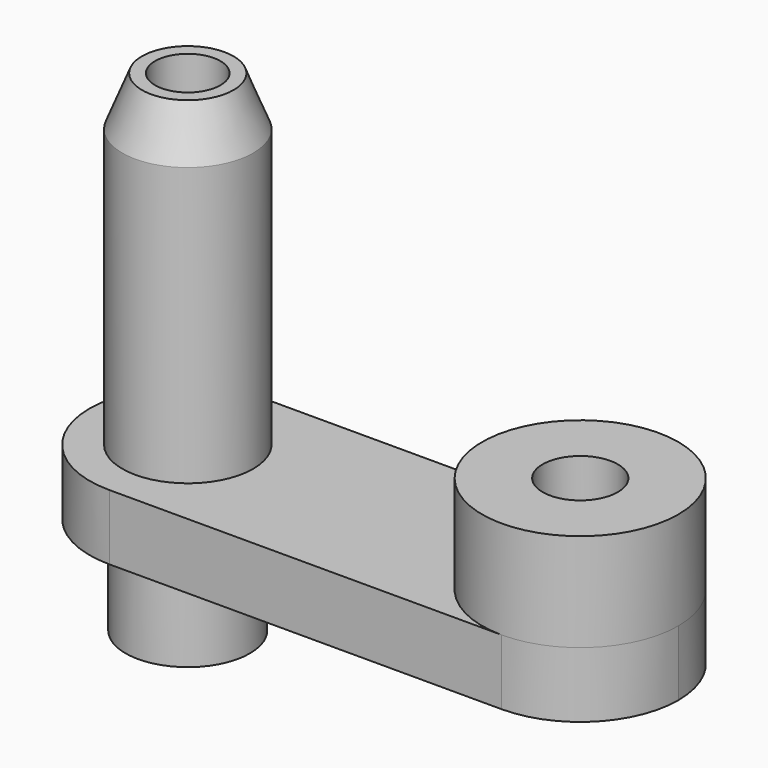
from build123d import *

# Parameters (mm, degrees)
F0_W      = 18
F0_H      = 6
F1_DEPTH  = 2
F2_R      = 3
F2_R_2    = 2
F3_DEPTH  = 10
F4_R      = 1
F4_R_2    = 1.15
F5_DEPTH  = 20
F6_SIZE2  = 1.5
F6_SIZE   = 0.6
F7_W      = 11.6012076614
F7_H      = 11.8295210414
F8_DEPTH  = 7
F9_R      = 2.9999
F10_R     = 1.9
F10_R_2   = 1
F11_DEPTH = 3


# Not quite as in the source:
# - a fillet or chamfer is up to 0.001 mm smaller than in the source, because OpenCascade refuses the exact size


with BuildPart() as f1:
    # F0 (on Top) → F1 (new body)
    with BuildSketch(Plane.XY):
        with Locations((1.8924829921, 0)):
            Rectangle(F0_W, F0_H)
    extrude(amount=F1_DEPTH)

    # F2 (on face) → F3 (join)
    with BuildSketch(Plane.XY.offset(2)):
        with Locations((7.8924829921, 0)):
            Circle(F2_R)
        with Locations((-4.1075170079, 0)):
            Circle(F2_R_2)
    extrude(amount=F3_DEPTH)

    # F4 (on face) → F5 (cut)
    with BuildSketch(Plane.XY.offset(12)):
        with Locations((-4.1075170079, 0)):
            Circle(F4_R)
        with Locations((7.8924829921, 0)):
            Circle(F4_R_2)
    extrude(amount=-F5_DEPTH, mode=Mode.SUBTRACT)

    # F6
    f6_edges = [f1.edges().sort_by_distance(p)[0] for p in [
        (-6.107517, 0, 12),
    ]]
    f6_side = f1.faces().sort_by_distance((-6.050948, 0, 12))[0]
    chamfer(f6_edges, length=F6_SIZE, length2=F6_SIZE2, reference=f6_side)

    # F7 (on face) → F8 (cut)
    with BuildSketch(Plane.XY.offset(12)):
        with Locations((7.5882198871, -0.5373002496)):
            Rectangle(F7_W, F7_H)
    extrude(amount=-F8_DEPTH, mode=Mode.SUBTRACT)

    # F9 (radius 3 in the source; OpenCascade refuses exactly that, so slightly less here)
    f9_edges = [f1.edges().sort_by_distance(p)[0] for p in [
        (10.892483, -3, 1),
        (10.892483, 3, 1),
        (-7.107517, 3, 1),
        (-7.107517, -3, 1),
    ]]
    fillet(f9_edges, radius=F9_R)

    # F10 (on face) → F11 (join)
    with BuildSketch(Plane(origin=(0, 0, 0), x_dir=(1, 0, 0), z_dir=(0, 0, -1))):
        with Locations((-4.1075170079, 0)):
            Circle(F10_R)
        with Locations((-4.1075170079, 0)):
            Circle(F10_R_2, mode=Mode.SUBTRACT)
    extrude(amount=F11_DEPTH)


solid = f1.part
